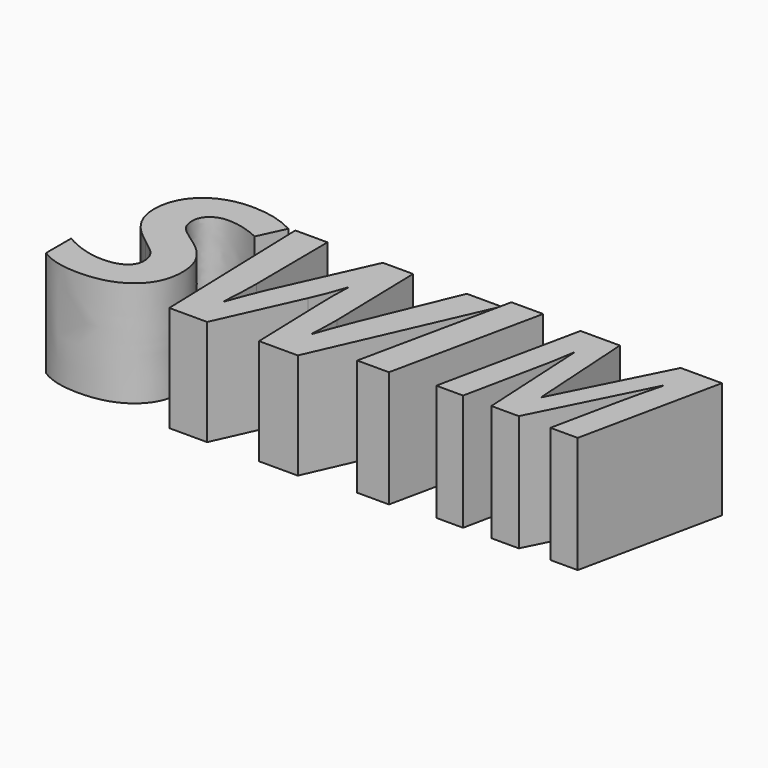
from build123d import *

# Parameters (mm, degrees)
F0_TEXT_SIZE = 44.2246531343
F1_DEPTH     = 20
F2_TEXT_SIZE = 43.3685692892
F3_DEPTH     = 20
F4_TEXT_SIZE = 40.2810498296
F5_DEPTH     = 22
F6_TEXT_SIZE = 37.7458804804
F7_DEPTH     = 22


# Not quite as in the source:
# - Text() gives the source's letters only with a copy of the font that has no kerning and outlines rounded to 1/6400 em; it was checked with that copy


with BuildPart() as f1:
    # F0 (on Top) → F1 (new body)
    with BuildSketch(Plane.XY):
        with Locations((-66.8646581471, -15.6653448357)):
            Text('S', F0_TEXT_SIZE, font='Open Sans', font_style=FontStyle.BOLDITALIC, text_align=(TextAlign.LEFT, TextAlign.BOTTOM))
    extrude(amount=F1_DEPTH)


with BuildPart() as f3:
    # F2 (on Top) → F3 (new body)
    with BuildSketch(Plane.XY):
        with Locations((-45.6521955158, -16.5213752713)):
            Text('W', F2_TEXT_SIZE, font='Open Sans', font_style=FontStyle.BOLDITALIC, text_align=(TextAlign.LEFT, TextAlign.BOTTOM))
    extrude(amount=F3_DEPTH)


with BuildPart() as f5:
    # F4 (on Top) → F5 (new body)
    with BuildSketch(Plane.XY):
        with Locations((-7.3012942448, -15.3124318458)):
            Text('I', F4_TEXT_SIZE, font='Open Sans', font_style=FontStyle.BOLDITALIC, text_align=(TextAlign.LEFT, TextAlign.BOTTOM))
    extrude(amount=F5_DEPTH)


with BuildPart() as f7:
    # F6 (on Top) → F7 (new body)
    with BuildSketch(Plane.XY):
        with Locations((6.8956636824, -14.2983654514)):
            Text('M', F6_TEXT_SIZE, font='Open Sans', font_style=FontStyle.BOLDITALIC, text_align=(TextAlign.LEFT, TextAlign.BOTTOM))
    extrude(amount=F7_DEPTH)


solid = Compound([f1.part, f3.part, f5.part, f7.part])
